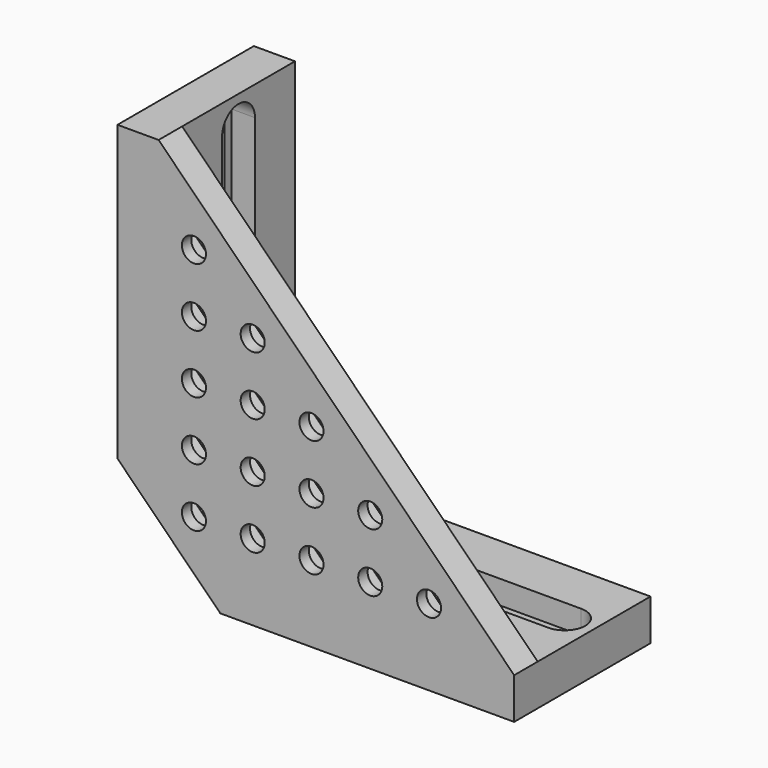
from build123d import *

# Parameters (mm, degrees)
F1_DEPTH  = 7
F2_DEPTH  = 3
F4_ANGLE  = 90
F8_ANGLE  = 180
F12_R     = 2.05
F13_DEPTH = 5
F14_DEPTH = 3


# Not quite as in the source:
# - a feature names something its author has since deleted; it is built from what else it names


with BuildPart() as f1:
    # F0 (on Top) → F1 (new body)
    with BuildSketch(Plane.XY):
        Polygon((29, 12), (-21, 12), (-21, -12), (0, -12), (29, -12), align=None)
        with BuildLine():
            ThreePointArc((-16, -11.5), (-19.5, -8), (-16, -4.5))
            Line((-16, -4.5), (0, -4.5))
            Line((0, -4.5), (24, -4.5))
            ThreePointArc((24, -4.5), (27.5, -8), (24, -11.5))
            Line((24, -11.5), (0, -11.5))
            Line((0, -11.5), (-16, -11.5))
        make_face(mode=Mode.SUBTRACT)
        with BuildLine():
            Line((0, -3.5), (-16, -3.5))
            ThreePointArc((-16, -3.5), (-19.5, 0), (-16, 3.5))
            Line((-16, 3.5), (0, 3.5))
            Line((0, 3.5), (24, 3.5))
            ThreePointArc((24, 3.5), (27.5, 0), (24, -3.5))
            Line((24, -3.5), (0, -3.5))
        make_face(mode=Mode.SUBTRACT)
        with BuildLine():
            Line((0, 4.5), (-16, 4.5))
            ThreePointArc((-16, 4.5), (-19.5, 8), (-16, 11.5))
            Line((-16, 11.5), (0, 11.5))
            Line((0, 11.5), (24, 11.5))
            ThreePointArc((24, 11.5), (27.5, 8), (24, 4.5))
            Line((24, 4.5), (0, 4.5))
        make_face(mode=Mode.SUBTRACT)
        with BuildLine():
            Line((0, -4.5), (-16, -4.5))
            ThreePointArc((-16, -4.5), (-19.5, -8), (-16, -11.5))
            Line((-16, -11.5), (0, -11.5))
            Line((0, -11.5), (24, -11.5))
            ThreePointArc((24, -11.5), (27.5, -8), (24, -4.5))
            Line((24, -4.5), (0, -4.5))
        make_face()
        with BuildLine():
            ThreePointArc((-16, -10.05), (-18.05, -8), (-16, -5.95))
            Line((-16, -5.95), (0, -5.95))
            Line((0, -5.95), (24, -5.95))
            ThreePointArc((24, -5.95), (26.05, -8), (24, -10.05))
            Line((24, -10.05), (0, -10.05))
            Line((0, -10.05), (-16, -10.05))
        make_face(mode=Mode.SUBTRACT)
        with BuildLine():
            ThreePointArc((-16, 11.5), (-19.5, 8), (-16, 4.5))
            Line((-16, 4.5), (0, 4.5))
            Line((0, 4.5), (24, 4.5))
            ThreePointArc((24, 4.5), (27.5, 8), (24, 11.5))
            Line((24, 11.5), (0, 11.5))
            Line((0, 11.5), (-16, 11.5))
        make_face()
        with BuildLine():
            Line((24, 5.95), (0, 5.95))
            Line((0, 5.95), (-16, 5.95))
            ThreePointArc((-16, 5.95), (-18.05, 8), (-16, 10.05))
            Line((-16, 10.05), (0, 10.05))
            Line((0, 10.05), (24, 10.05))
            ThreePointArc((24, 10.05), (26.05, 8), (24, 5.95))
        make_face(mode=Mode.SUBTRACT)
        with BuildLine():
            Line((0, -5.95), (-16, -5.95))
            ThreePointArc((-16, -5.95), (-18.05, -8), (-16, -10.05))
            Line((-16, -10.05), (0, -10.05))
            Line((0, -10.05), (24, -10.05))
            ThreePointArc((24, -10.05), (26.05, -8), (24, -5.95))
            Line((24, -5.95), (0, -5.95))
        make_face()
        with BuildLine():
            Line((-16, 5.95), (0, 5.95))
            Line((0, 5.95), (24, 5.95))
            ThreePointArc((24, 5.95), (26.05, 8), (24, 10.05))
            Line((24, 10.05), (0, 10.05))
            Line((0, 10.05), (-16, 10.05))
            ThreePointArc((-16, 10.05), (-18.05, 8), (-16, 5.95))
        make_face()
    extrude(amount=F1_DEPTH)

    # F0 (on Top) → F2 (join)
    with BuildSketch(Plane.XY):
        with BuildLine():
            ThreePointArc((-16, 3.5), (-19.5, 0), (-16, -3.5))
            Line((-16, -3.5), (0, -3.5))
            Line((0, -3.5), (24, -3.5))
            ThreePointArc((24, -3.5), (27.5, 0), (24, 3.5))
            Line((24, 3.5), (0, 3.5))
            Line((0, 3.5), (-16, 3.5))
        make_face()
        with BuildLine():
            Line((0, -2.05), (-16, -2.05))
            ThreePointArc((-16, -2.05), (-18.05, 0), (-16, 2.05))
            Line((-16, 2.05), (0, 2.05))
            Line((0, 2.05), (24, 2.05))
            ThreePointArc((24, 2.05), (26.05, 0), (24, -2.05))
            Line((24, -2.05), (0, -2.05))
        make_face(mode=Mode.SUBTRACT)
    extrude(amount=F2_DEPTH)


with BuildPart() as f4_1:
    # F4: copy of F1
    add(f1.part.rotate(Axis((-21, 0, 3.5), (0, -1, 0)), F4_ANGLE))


with BuildPart() as f4_1_1:
    # F8: moved
    add(f4_1.part.rotate(Axis((-21, 0, 28.5), (0, 0, 1)), F8_ANGLE))


with BuildPart() as f4_1_2:
    # F9: moved
    add(f4_1_1.part.moved(Location((0, 0, 14))))


with BuildPart() as f4_1_3:
    # F10: moved
    add(f4_1_2.part.moved(Location((-14, 0, 0))))


with BuildPart() as f1_1:
    add(f1.part)

    add(f4_1_3.part)  # F13 merges F4_1
    # F12 (on 3pt) → F13 (join)
    with BuildSketch(Plane.XZ.offset(12)):
        Polygon((-38.5, 17.5), (-21, 0), (29, 0), (29, 7), (-31.5, 67.5), (-38.5, 67.5), align=None)
        Polygon((-29.3563439923, 11.9720831325), (-28.3210678119, 15.8357864376), (-24.4573645067, 16.871062618), (-21.628937382, 14.0426354933), (-22.6642135624, 10.1789321881), (-26.5279168675, 9.1436560077), align=None, mode=Mode.SUBTRACT)
        Polygon((-19.3563439923, 11.9720831325), (-18.3210678119, 15.8357864376), (-14.4573645067, 16.871062618), (-11.628937382, 14.0426354933), (-12.6642135624, 10.1789321881), (-16.5279168675, 9.1436560077), align=None, mode=Mode.SUBTRACT)
        Polygon((-9.3563439923, 11.9720831325), (-8.3210678119, 15.8357864376), (-4.4573645067, 16.871062618), (-1.628937382, 14.0426354933), (-2.6642135624, 10.1789321881), (-6.5279168675, 9.1436560077), align=None, mode=Mode.SUBTRACT)
        Polygon((-29.3563439923, 21.9720831325), (-28.3210678119, 25.8357864376), (-24.4573645067, 26.871062618), (-21.628937382, 24.0426354933), (-22.6642135624, 20.1789321881), (-26.5279168675, 19.1436560077), align=None, mode=Mode.SUBTRACT)
        Polygon((-29.3563439923, 31.9720831325), (-28.3210678119, 35.8357864376), (-24.4573645067, 36.871062618), (-21.628937382, 34.0426354933), (-22.6642135624, 30.1789321881), (-26.5279168675, 29.1436560077), align=None, mode=Mode.SUBTRACT)
        Polygon((-19.3563439923, 21.9720831325), (-18.3210678119, 25.8357864376), (-14.4573645067, 26.871062618), (-11.628937382, 24.0426354933), (-12.6642135624, 20.1789321881), (-16.5279168675, 19.1436560077), align=None, mode=Mode.SUBTRACT)
        Polygon((-9.3563439923, 21.9720831325), (-8.3210678119, 25.8357864376), (-4.4573645067, 26.871062618), (-1.628937382, 24.0426354933), (-2.6642135624, 20.1789321881), (-6.5279168675, 19.1436560077), align=None, mode=Mode.SUBTRACT)
        Polygon((-19.3563439923, 31.9720831325), (-18.3210678119, 35.8357864376), (-14.4573645067, 36.871062618), (-11.628937382, 34.0426354933), (-12.6642135624, 30.1789321881), (-16.5279168675, 29.1436560077), align=None, mode=Mode.SUBTRACT)
        Polygon((-9.3563439923, 31.9720831325), (-8.3210678119, 35.8357864376), (-4.4573645067, 36.871062618), (-1.628937382, 34.0426354933), (-2.6642135624, 30.1789321881), (-6.5279168675, 29.1436560077), align=None, mode=Mode.SUBTRACT)
        Polygon((0.6436560077, 11.9720831325), (1.6789321881, 15.8357864376), (5.5426354933, 16.871062618), (8.371062618, 14.0426354933), (7.3357864376, 10.1789321881), (3.4720831325, 9.1436560077), align=None, mode=Mode.SUBTRACT)
        Polygon((10.6436560077, 11.9720831325), (11.6789321881, 15.8357864376), (15.5426354933, 16.871062618), (18.371062618, 14.0426354933), (17.3357864376, 10.1789321881), (13.4720831325, 9.1436560077), align=None, mode=Mode.SUBTRACT)
        Polygon((0.6436560077, 21.9720831325), (1.6789321881, 25.8357864376), (5.5426354933, 26.871062618), (8.371062618, 24.0426354933), (7.3357864376, 20.1789321881), (3.4720831325, 19.1436560077), align=None, mode=Mode.SUBTRACT)
        Polygon((-29.3563439923, 41.9720831325), (-28.3210678119, 45.8357864376), (-24.4573645067, 46.871062618), (-21.628937382, 44.0426354933), (-22.6642135624, 40.1789321881), (-26.5279168675, 39.1436560077), align=None, mode=Mode.SUBTRACT)
        Polygon((-19.3563439923, 41.9720831325), (-18.3210678119, 45.8357864376), (-14.4573645067, 46.871062618), (-11.628937382, 44.0426354933), (-12.6642135624, 40.1789321881), (-16.5279168675, 39.1436560077), align=None, mode=Mode.SUBTRACT)
        Polygon((-26.5279168675, 49.1436560077), (-29.3563439923, 51.9720831325), (-28.3210678119, 55.8357864376), (-24.4573645067, 56.871062618), (-21.628937382, 54.0426354933), (-22.6642135624, 50.1789321881), align=None, mode=Mode.SUBTRACT)
        Polygon((-4.4573645067, 36.871062618), (-8.3210678119, 35.8357864376), (-9.3563439923, 31.9720831325), (-6.5279168675, 29.1436560077), (-2.6642135624, 30.1789321881), (-1.628937382, 34.0426354933), align=None)
        with Locations((-5.4926406871, 33.0073593129)):
            Circle(F12_R, mode=Mode.SUBTRACT)
        Polygon((-14.4573645067, 46.871062618), (-18.3210678119, 45.8357864376), (-19.3563439923, 41.9720831325), (-16.5279168675, 39.1436560077), (-12.6642135624, 40.1789321881), (-11.628937382, 44.0426354933), align=None)
        with Locations((-15.4926406871, 43.0073593129)):
            Circle(F12_R, mode=Mode.SUBTRACT)
        Polygon((-14.4573645067, 36.871062618), (-18.3210678119, 35.8357864376), (-19.3563439923, 31.9720831325), (-16.5279168675, 29.1436560077), (-12.6642135624, 30.1789321881), (-11.628937382, 34.0426354933), align=None)
        with Locations((-15.4926406871, 33.0073593129)):
            Circle(F12_R, mode=Mode.SUBTRACT)
        Polygon((-14.4573645067, 26.871062618), (-18.3210678119, 25.8357864376), (-19.3563439923, 21.9720831325), (-16.5279168675, 19.1436560077), (-12.6642135624, 20.1789321881), (-11.628937382, 24.0426354933), align=None)
        with Locations((-15.4926406871, 23.0073593129)):
            Circle(F12_R, mode=Mode.SUBTRACT)
        Polygon((-4.4573645067, 26.871062618), (-8.3210678119, 25.8357864376), (-9.3563439923, 21.9720831325), (-6.5279168675, 19.1436560077), (-2.6642135624, 20.1789321881), (-1.628937382, 24.0426354933), align=None)
        with Locations((-5.4926406871, 23.0073593129)):
            Circle(F12_R, mode=Mode.SUBTRACT)
        Polygon((5.5426354933, 26.871062618), (1.6789321881, 25.8357864376), (0.6436560077, 21.9720831325), (3.4720831325, 19.1436560077), (7.3357864376, 20.1789321881), (8.371062618, 24.0426354933), align=None)
        with Locations((4.5073593129, 23.0073593129)):
            Circle(F12_R, mode=Mode.SUBTRACT)
        Polygon((-28.3210678119, 55.8357864376), (-29.3563439923, 51.9720831325), (-26.5279168675, 49.1436560077), (-22.6642135624, 50.1789321881), (-21.628937382, 54.0426354933), (-24.4573645067, 56.871062618), align=None)
        with Locations((-25.4926406871, 53.0073593129)):
            Circle(F12_R, mode=Mode.SUBTRACT)
        Polygon((-24.4573645067, 46.871062618), (-28.3210678119, 45.8357864376), (-29.3563439923, 41.9720831325), (-26.5279168675, 39.1436560077), (-22.6642135624, 40.1789321881), (-21.628937382, 44.0426354933), align=None)
        with Locations((-25.4926406871, 43.0073593129)):
            Circle(F12_R, mode=Mode.SUBTRACT)
        Polygon((-24.4573645067, 36.871062618), (-28.3210678119, 35.8357864376), (-29.3563439923, 31.9720831325), (-26.5279168675, 29.1436560077), (-22.6642135624, 30.1789321881), (-21.628937382, 34.0426354933), align=None)
        with Locations((-25.4926406871, 33.0073593129)):
            Circle(F12_R, mode=Mode.SUBTRACT)
        Polygon((-24.4573645067, 26.871062618), (-28.3210678119, 25.8357864376), (-29.3563439923, 21.9720831325), (-26.5279168675, 19.1436560077), (-22.6642135624, 20.1789321881), (-21.628937382, 24.0426354933), align=None)
        with Locations((-25.4926406871, 23.0073593129)):
            Circle(F12_R, mode=Mode.SUBTRACT)
        Polygon((-24.4573645067, 16.871062618), (-28.3210678119, 15.8357864376), (-29.3563439923, 11.9720831325), (-26.5279168675, 9.1436560077), (-22.6642135624, 10.1789321881), (-21.628937382, 14.0426354933), align=None)
        with Locations((-25.4926406871, 13.0073593129)):
            Circle(F12_R, mode=Mode.SUBTRACT)
        Polygon((-14.4573645067, 16.871062618), (-18.3210678119, 15.8357864376), (-19.3563439923, 11.9720831325), (-16.5279168675, 9.1436560077), (-12.6642135624, 10.1789321881), (-11.628937382, 14.0426354933), align=None)
        with Locations((-15.4926406871, 13.0073593129)):
            Circle(F12_R, mode=Mode.SUBTRACT)
        Polygon((-4.4573645067, 16.871062618), (-8.3210678119, 15.8357864376), (-9.3563439923, 11.9720831325), (-6.5279168675, 9.1436560077), (-2.6642135624, 10.1789321881), (-1.628937382, 14.0426354933), align=None)
        with Locations((-5.4926406871, 13.0073593129)):
            Circle(F12_R, mode=Mode.SUBTRACT)
        Polygon((5.5426354933, 16.871062618), (1.6789321881, 15.8357864376), (0.6436560077, 11.9720831325), (3.4720831325, 9.1436560077), (7.3357864376, 10.1789321881), (8.371062618, 14.0426354933), align=None)
        with Locations((4.5073593129, 13.0073593129)):
            Circle(F12_R, mode=Mode.SUBTRACT)
        Polygon((15.5426354933, 16.871062618), (11.6789321881, 15.8357864376), (10.6436560077, 11.9720831325), (13.4720831325, 9.1436560077), (17.3357864376, 10.1789321881), (18.371062618, 14.0426354933), align=None)
        with Locations((14.5073593129, 13.0073593129)):
            Circle(F12_R, mode=Mode.SUBTRACT)
    extrude(amount=F13_DEPTH)

    # F12 (on 3pt) → F14 (cut)
    with BuildSketch(Plane.XZ.offset(12)):
        Polygon((-4.4573645067, 36.871062618), (-8.3210678119, 35.8357864376), (-9.3563439923, 31.9720831325), (-6.5279168675, 29.1436560077), (-2.6642135624, 30.1789321881), (-1.628937382, 34.0426354933), align=None)
        with Locations((-5.4926406871, 33.0073593129)):
            Circle(F12_R, mode=Mode.SUBTRACT)
        Polygon((5.5426354933, 26.871062618), (1.6789321881, 25.8357864376), (0.6436560077, 21.9720831325), (3.4720831325, 19.1436560077), (7.3357864376, 20.1789321881), (8.371062618, 24.0426354933), align=None)
        with Locations((4.5073593129, 23.0073593129)):
            Circle(F12_R, mode=Mode.SUBTRACT)
        Polygon((-4.4573645067, 26.871062618), (-8.3210678119, 25.8357864376), (-9.3563439923, 21.9720831325), (-6.5279168675, 19.1436560077), (-2.6642135624, 20.1789321881), (-1.628937382, 24.0426354933), align=None)
        with Locations((-5.4926406871, 23.0073593129)):
            Circle(F12_R, mode=Mode.SUBTRACT)
        Polygon((-14.4573645067, 26.871062618), (-18.3210678119, 25.8357864376), (-19.3563439923, 21.9720831325), (-16.5279168675, 19.1436560077), (-12.6642135624, 20.1789321881), (-11.628937382, 24.0426354933), align=None)
        with Locations((-15.4926406871, 23.0073593129)):
            Circle(F12_R, mode=Mode.SUBTRACT)
        Polygon((-14.4573645067, 36.871062618), (-18.3210678119, 35.8357864376), (-19.3563439923, 31.9720831325), (-16.5279168675, 29.1436560077), (-12.6642135624, 30.1789321881), (-11.628937382, 34.0426354933), align=None)
        with Locations((-15.4926406871, 33.0073593129)):
            Circle(F12_R, mode=Mode.SUBTRACT)
        Polygon((-14.4573645067, 46.871062618), (-18.3210678119, 45.8357864376), (-19.3563439923, 41.9720831325), (-16.5279168675, 39.1436560077), (-12.6642135624, 40.1789321881), (-11.628937382, 44.0426354933), align=None)
        with Locations((-15.4926406871, 43.0073593129)):
            Circle(F12_R, mode=Mode.SUBTRACT)
        Polygon((15.5426354933, 16.871062618), (11.6789321881, 15.8357864376), (10.6436560077, 11.9720831325), (13.4720831325, 9.1436560077), (17.3357864376, 10.1789321881), (18.371062618, 14.0426354933), align=None)
        with Locations((14.5073593129, 13.0073593129)):
            Circle(F12_R, mode=Mode.SUBTRACT)
        Polygon((5.5426354933, 16.871062618), (1.6789321881, 15.8357864376), (0.6436560077, 11.9720831325), (3.4720831325, 9.1436560077), (7.3357864376, 10.1789321881), (8.371062618, 14.0426354933), align=None)
        with Locations((4.5073593129, 13.0073593129)):
            Circle(F12_R, mode=Mode.SUBTRACT)
        Polygon((-4.4573645067, 16.871062618), (-8.3210678119, 15.8357864376), (-9.3563439923, 11.9720831325), (-6.5279168675, 9.1436560077), (-2.6642135624, 10.1789321881), (-1.628937382, 14.0426354933), align=None)
        with Locations((-5.4926406871, 13.0073593129)):
            Circle(F12_R, mode=Mode.SUBTRACT)
        Polygon((-14.4573645067, 16.871062618), (-18.3210678119, 15.8357864376), (-19.3563439923, 11.9720831325), (-16.5279168675, 9.1436560077), (-12.6642135624, 10.1789321881), (-11.628937382, 14.0426354933), align=None)
        with Locations((-15.4926406871, 13.0073593129)):
            Circle(F12_R, mode=Mode.SUBTRACT)
        Polygon((-24.4573645067, 16.871062618), (-28.3210678119, 15.8357864376), (-29.3563439923, 11.9720831325), (-26.5279168675, 9.1436560077), (-22.6642135624, 10.1789321881), (-21.628937382, 14.0426354933), align=None)
        with Locations((-25.4926406871, 13.0073593129)):
            Circle(F12_R, mode=Mode.SUBTRACT)
        Polygon((-24.4573645067, 26.871062618), (-28.3210678119, 25.8357864376), (-29.3563439923, 21.9720831325), (-26.5279168675, 19.1436560077), (-22.6642135624, 20.1789321881), (-21.628937382, 24.0426354933), align=None)
        with Locations((-25.4926406871, 23.0073593129)):
            Circle(F12_R, mode=Mode.SUBTRACT)
        Polygon((-24.4573645067, 36.871062618), (-28.3210678119, 35.8357864376), (-29.3563439923, 31.9720831325), (-26.5279168675, 29.1436560077), (-22.6642135624, 30.1789321881), (-21.628937382, 34.0426354933), align=None)
        with Locations((-25.4926406871, 33.0073593129)):
            Circle(F12_R, mode=Mode.SUBTRACT)
        Polygon((-24.4573645067, 46.871062618), (-28.3210678119, 45.8357864376), (-29.3563439923, 41.9720831325), (-26.5279168675, 39.1436560077), (-22.6642135624, 40.1789321881), (-21.628937382, 44.0426354933), align=None)
        with Locations((-25.4926406871, 43.0073593129)):
            Circle(F12_R, mode=Mode.SUBTRACT)
        Polygon((-28.3210678119, 55.8357864376), (-29.3563439923, 51.9720831325), (-26.5279168675, 49.1436560077), (-22.6642135624, 50.1789321881), (-21.628937382, 54.0426354933), (-24.4573645067, 56.871062618), align=None)
        with Locations((-25.4926406871, 53.0073593129)):
            Circle(F12_R, mode=Mode.SUBTRACT)
    extrude(amount=F14_DEPTH, mode=Mode.SUBTRACT)


solid = f1_1.part
